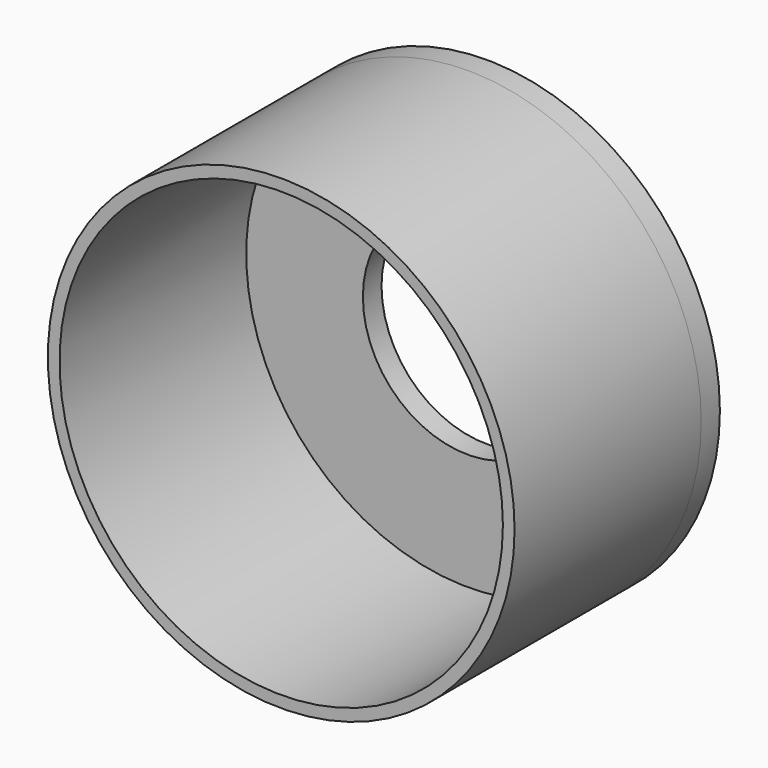
from build123d import *

# Parameters (mm, degrees)
F0_R     = 50
F1_DEPTH = 5
F2_R     = 50
F2_R_2   = 47.5
F3_DEPTH = 50
F4_R     = 22.5
F6_DEPTH = 55.001


# Not quite as in the source:
# - the program builds the solid bodies; features that only make, move or delete a surface that nothing else refers to are left out


with BuildPart() as f1:
    # F0 (on Front) → F1 (new body)
    with BuildSketch(Plane.XZ):
        Circle(F0_R)
    extrude(amount=-F1_DEPTH)

    # F2 (on Front) → F3 (join)
    with BuildSketch(Plane.XZ):
        Circle(F2_R)
        Circle(F2_R_2, mode=Mode.SUBTRACT)
    extrude(amount=F3_DEPTH)

    # F4 (on face) → F6 (cut, through all)
    with BuildSketch(Plane(origin=(0, 5, 0), x_dir=(-1, 0, 0), z_dir=(0, 1, 0))):
        Circle(F4_R)
    extrude(amount=-F6_DEPTH, mode=Mode.SUBTRACT)


solid = f1.part
